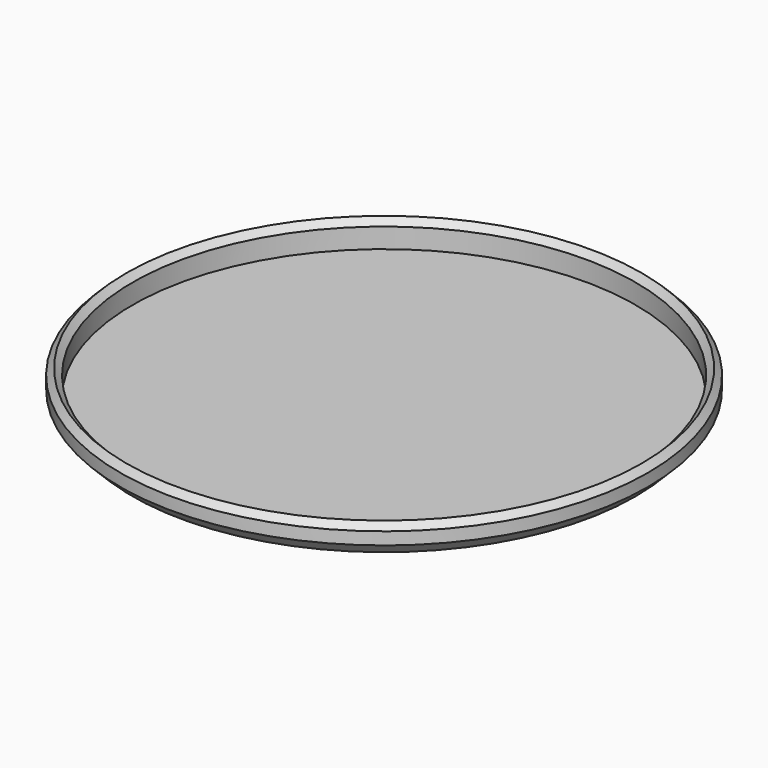
from build123d import *

# Parameters (mm, degrees)
F0_R     = 40.5
F1_DEPTH = 0.8
F0_R_2   = 42.5
F2_DEPTH = 5
F3_SIZE  = 2
F4_SIZE  = 0.99999


# Not quite as in the source:
# - a fillet or chamfer is up to 0.001 mm smaller than in the source, because OpenCascade refuses the exact size


with BuildPart() as f1:
    # F0 (on Top) → F1 (new body)
    with BuildSketch(Plane.XY):
        Circle(F0_R)
    extrude(amount=F1_DEPTH)

    # F0 (on Top) → F2 (join)
    with BuildSketch(Plane.XY):
        Circle(F0_R_2)
        Circle(F0_R, mode=Mode.SUBTRACT)
    extrude(amount=F2_DEPTH)

    # F3
    f3_edges = [f1.edges().sort_by_distance(p)[0] for p in [
        (-42.5, 0, 0),
    ]]
    chamfer(f3_edges, length=F3_SIZE)

    # F4 (size 1 in the source; OpenCascade refuses exactly that, so slightly less here)
    f4_edges = [f1.edges().sort_by_distance(p)[0] for p in [
        (-40.5, 0, 5),
        (-42.5, 0, 5),
    ]]
    chamfer(f4_edges, length=F4_SIZE)


solid = f1.part
